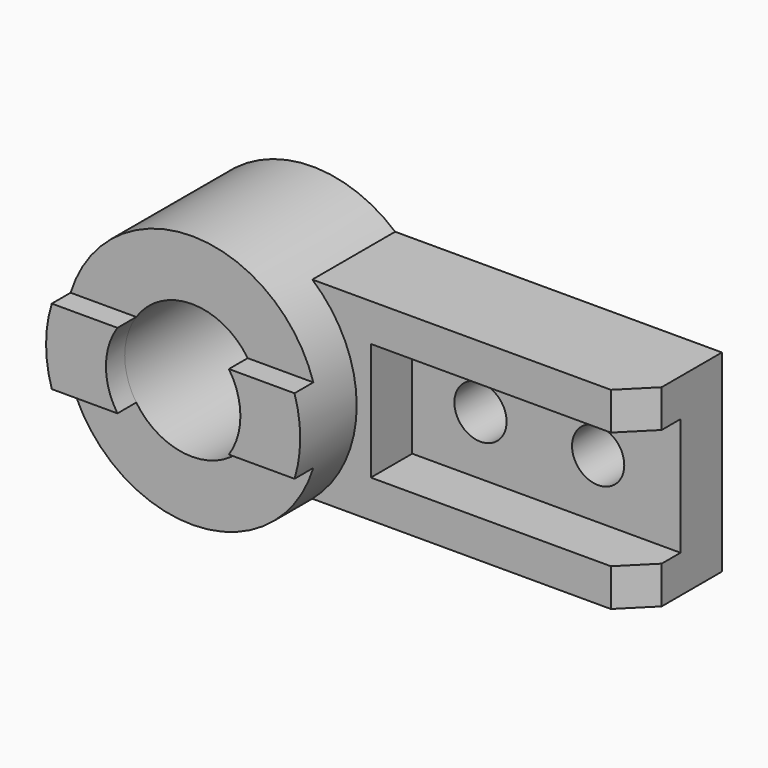
from build123d import *

# Parameters (mm, degrees)
F0_R     = 28.575
F1_DEPTH = 64
F0_R_2   = 11.1
F2_DEPTH = 44
F3_W     = 114
F3_H     = 50
F4_DEPTH = 22
F5_SIZE  = 12
F7_DEPTH = 10
F8_SIZE  = 12


# Not quite as in the source:
# - after a boolean that leaves OpenCascade's solid faulty, fix() repairs it


with BuildPart() as f1:
    # F0 (on Front) → F1 (new body)
    with BuildSketch(Plane.XZ):
        with BuildLine():
            ThreePointArc((35.1425667816, -41), (49.0596504584, -22.5643678594), (54, 0))
            ThreePointArc((54, 0), (49.0596504584, 22.5643678594), (35.1425667816, 41))
            ThreePointArc((35.1425667816, 41), (-54, 0), (35.1425667816, -41))
        make_face()
        Circle(F0_R, mode=Mode.SUBTRACT)
    extrude(amount=F1_DEPTH)

    # F0 (on Front) → F2 (join)
    with BuildSketch(Plane.XZ):
        with BuildLine():
            ThreePointArc((35.1425667816, 41), (49.0596504584, 22.5643678594), (54, 0))
            ThreePointArc((54, 0), (49.0596504584, -22.5643678594), (35.1425667816, -41))
            Line((35.1425667816, -41), (174, -41))
            Line((174, -41), (174, 41))
            Line((174, 41), (35.1425667816, 41))
        make_face()
        with Locations((89, 0)):
            Circle(F0_R_2, mode=Mode.SUBTRACT)
        with Locations((139, 0)):
            Circle(F0_R_2, mode=Mode.SUBTRACT)
    extrude(amount=F2_DEPTH)

    # F3 (on face) → F4 (cut)
    with BuildSketch(Plane.XZ.offset(44)):
        with Locations((117, 0)):
            Rectangle(F3_W, F3_H)
    extrude(amount=-F4_DEPTH, mode=Mode.SUBTRACT)

    # F5
    f5_edges = [f1.edges().sort_by_distance(p)[0] for p in [
        (174, -44, -33),
    ]]
    chamfer(f5_edges, length=F5_SIZE)

    # F6 (on face) → F7 (join)
    with BuildSketch(Plane.XZ.offset(64)):
        with BuildLine():
            Line((-23.6755279772, 16), (-51.5751878329, 16))
            ThreePointArc((-51.5751878329, 16), (-54, 0), (-51.5751878329, -16))
            Line((-51.5751878329, -16), (-23.6755279772, -16))
            ThreePointArc((-23.6755279772, -16), (-28.575, 0), (-23.6755279772, 16))
        make_face()
        with BuildLine():
            Line((51.5751878329, 16), (23.6755279772, 16))
            ThreePointArc((23.6755279772, 16), (28.575, 0), (23.6755279772, -16))
            Line((23.6755279772, -16), (51.5751878329, -16))
            ThreePointArc((51.5751878329, -16), (54, 0), (51.5751878329, 16))
        make_face()
    extrude(amount=F7_DEPTH)

    add(f1.part.fix(), mode=Mode.REPLACE)

    # F8
    f8_edges = [f1.edges().sort_by_distance(p)[0] for p in [
        (174, -44, 33),
    ]]
    chamfer(f8_edges, length=F8_SIZE)


solid = f1.part
